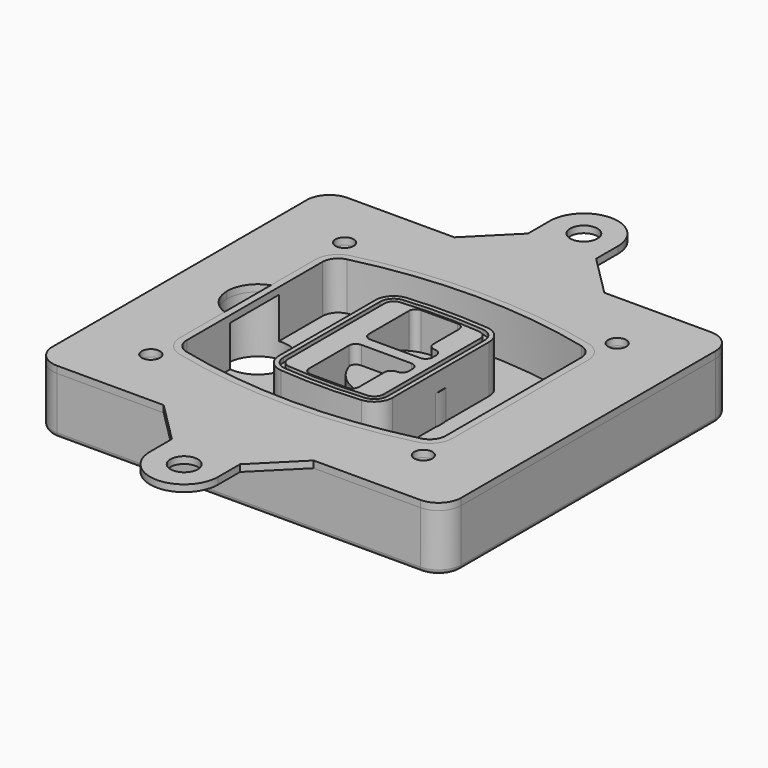
from build123d import *

# Parameters (mm, degrees)
F0_R      = 4
F1_DEPTH  = 25
F2_DEPTH  = 3
F3_DEPTH  = 18
F5_DEPTH  = 21
F6_DEPTH  = 2
F8_DEPTH  = 20
F9_DEPTH  = 16
F10_DEPTH = 25
F7_R      = 6
F7_R_2    = 4
F11_DEPTH = 6
F13_DEPTH = 9
F15_R     = 2
F16_R     = 6
F16_R_2   = 4
F17_DEPTH = 3


# Not quite as in the source:
# - a feature of the source that left no trace in its solid (it failed there, or was rolled back) is left out
# - a feature names something its author has since deleted; it is built from what else it names


with BuildPart() as f1:
    # F0 (on Top) → F1 (new body)
    with BuildSketch(Plane.XY):
        with BuildLine():
            ThreePointArc((-90, -70), (-87.0710678119, -77.0710678119), (-80, -80))
            Line((-80, -80), (80, -80))
            ThreePointArc((80, -80), (87.0710678119, -77.0710678119), (90, -70))
            Line((90, -70), (90, 70))
            ThreePointArc((90, 70), (87.0710678119, 77.0710678119), (80, 80))
            Line((80, 80), (-80, 80))
            ThreePointArc((-80, 80), (-87.0710678119, 77.0710678119), (-90, 70))
            Line((-90, 70), (-90, -70))
        make_face()
        with Locations((-60, -53.3333333333)):
            Circle(F0_R, mode=Mode.SUBTRACT)
        with Locations((60, -53.3333333333)):
            Circle(F0_R, mode=Mode.SUBTRACT)
        with Locations((-60, 53.3333333333)):
            Circle(F0_R, mode=Mode.SUBTRACT)
        with BuildLine():
            ThreePointArc((-64, 37.2990447398), (-61.0143011354, 45.9411029726), (-53.3306899286, 50.8970778549))
            ThreePointArc((-53.3306899286, 50.8970778549), (0, 57.3333333333), (53.3306899286, 50.8970778549))
            ThreePointArc((53.3306899286, 50.8970778549), (61.0143011354, 45.9411029726), (64, 37.2990447398))
            Line((64, 37.2990447398), (64, -37.2990447398))
            ThreePointArc((64, -37.2990447398), (61.0143011354, -45.9411029726), (53.3306899286, -50.8970778549))
            ThreePointArc((53.3306899286, -50.8970778549), (0, -57.3333333333), (-53.3306899286, -50.8970778549))
            ThreePointArc((-53.3306899286, -50.8970778549), (-61.0143011354, -45.9411029726), (-64, -37.2990447398))
            Line((-64, -37.2990447398), (-64, 37.2990447398))
        make_face(mode=Mode.SUBTRACT)
        with Locations((60, 53.3333333333)):
            Circle(F0_R, mode=Mode.SUBTRACT)
        with BuildLine():
            ThreePointArc((53.3306899286, 50.8970778549), (0, 57.3333333333), (-53.3306899286, 50.8970778549))
            ThreePointArc((-53.3306899286, 50.8970778549), (-61.0143011354, 45.9411029726), (-64, 37.2990447398))
            Line((-64, 37.2990447398), (-64, -37.2990447398))
            ThreePointArc((-64, -37.2990447398), (-61.0143011354, -45.9411029726), (-53.3306899286, -50.8970778549))
            ThreePointArc((-53.3306899286, -50.8970778549), (0, -57.3333333333), (53.3306899286, -50.8970778549))
            ThreePointArc((53.3306899286, -50.8970778549), (61.0143011354, -45.9411029726), (64, -37.2990447398))
            Line((64, -37.2990447398), (64, 37.2990447398))
            ThreePointArc((64, 37.2990447398), (61.0143011354, 45.9411029726), (53.3306899286, 50.8970778549))
        make_face()
        with BuildLine():
            Line((-60, -37.2990447398), (-60, 37.2990447398))
            ThreePointArc((-60, 37.2990447398), (-57.8673579538, 43.4719434775), (-52.3790642347, 47.0119255363))
            ThreePointArc((-52.3790642347, 47.0119255363), (0, 53.3333333333), (52.3790642347, 47.0119255363))
            ThreePointArc((52.3790642347, 47.0119255363), (57.8673579538, 43.4719434775), (60, 37.2990447398))
            Line((60, 37.2990447398), (60, -37.2990447398))
            ThreePointArc((60, -37.2990447398), (57.8673579538, -43.4719434775), (52.3790642347, -47.0119255363))
            ThreePointArc((52.3790642347, -47.0119255363), (0, -53.3333333333), (-52.3790642347, -47.0119255363))
            ThreePointArc((-52.3790642347, -47.0119255363), (-57.8673579538, -43.4719434775), (-60, -37.2990447398))
        make_face(mode=Mode.SUBTRACT)
        with BuildLine():
            ThreePointArc((-52.3790642347, 47.0119255363), (-57.8673579538, 43.4719434775), (-60, 37.2990447398))
            Line((-60, 37.2990447398), (-60, -37.2990447398))
            ThreePointArc((-60, -37.2990447398), (-57.8673579538, -43.4719434775), (-52.3790642347, -47.0119255363))
            ThreePointArc((-52.3790642347, -47.0119255363), (0, -53.3333333333), (52.3790642347, -47.0119255363))
            ThreePointArc((52.3790642347, -47.0119255363), (57.8673579538, -43.4719434775), (60, -37.2990447398))
            Line((60, -37.2990447398), (60, 37.2990447398))
            ThreePointArc((60, 37.2990447398), (57.8673579538, 43.4719434775), (52.3790642347, 47.0119255363))
            ThreePointArc((52.3790642347, 47.0119255363), (0, 53.3333333333), (-52.3790642347, 47.0119255363))
        make_face()
        with BuildLine():
            ThreePointArc((51.6653449643, 44.0980612973), (55.5071505677, 41.6200738562), (57, 37.2990447398))
            Line((57, 37.2990447398), (57, -37.2990447398))
            ThreePointArc((57, -37.2990447398), (55.5071505677, -41.6200738562), (51.6653449643, -44.0980612973))
            ThreePointArc((51.6653449643, -44.0980612973), (0, -50.3333333333), (-51.6653449643, -44.0980612973))
            ThreePointArc((-51.6653449643, -44.0980612973), (-55.5071505677, -41.6200738562), (-57, -37.2990447398))
            Line((-57, -37.2990447398), (-57, 37.2990447398))
            ThreePointArc((-57, 37.2990447398), (-55.5071505677, 41.6200738562), (-51.6653449643, 44.0980612973))
            ThreePointArc((-51.6653449643, 44.0980612973), (0, 50.3333333333), (51.6653449643, 44.0980612973))
        make_face(mode=Mode.SUBTRACT)
        with BuildLine():
            Line((57, -37.2990447398), (57, 37.2990447398))
            ThreePointArc((57, 37.2990447398), (55.5071505677, 41.6200738562), (51.6653449643, 44.0980612973))
            ThreePointArc((51.6653449643, 44.0980612973), (0, 50.3333333333), (-51.6653449643, 44.0980612973))
            ThreePointArc((-51.6653449643, 44.0980612973), (-55.5071505677, 41.6200738562), (-57, 37.2990447398))
            Line((-57, 37.2990447398), (-57, -37.2990447398))
            ThreePointArc((-57, -37.2990447398), (-55.5071505677, -41.6200738562), (-51.6653449643, -44.0980612973))
            ThreePointArc((-51.6653449643, -44.0980612973), (0, -50.3333333333), (51.6653449643, -44.0980612973))
            ThreePointArc((51.6653449643, -44.0980612973), (55.5071505677, -41.6200738562), (57, -37.2990447398))
        make_face()
    extrude(amount=-F1_DEPTH)

    # F0 (on Top) → F2 (join)
    with BuildSketch(Plane.XY):
        with BuildLine():
            ThreePointArc((-52.3790642347, 47.0119255363), (-57.8673579538, 43.4719434775), (-60, 37.2990447398))
            Line((-60, 37.2990447398), (-60, -37.2990447398))
            ThreePointArc((-60, -37.2990447398), (-57.8673579538, -43.4719434775), (-52.3790642347, -47.0119255363))
            ThreePointArc((-52.3790642347, -47.0119255363), (0, -53.3333333333), (52.3790642347, -47.0119255363))
            ThreePointArc((52.3790642347, -47.0119255363), (57.8673579538, -43.4719434775), (60, -37.2990447398))
            Line((60, -37.2990447398), (60, 37.2990447398))
            ThreePointArc((60, 37.2990447398), (57.8673579538, 43.4719434775), (52.3790642347, 47.0119255363))
            ThreePointArc((52.3790642347, 47.0119255363), (0, 53.3333333333), (-52.3790642347, 47.0119255363))
        make_face()
        with BuildLine():
            ThreePointArc((51.6653449643, 44.0980612973), (55.5071505677, 41.6200738562), (57, 37.2990447398))
            Line((57, 37.2990447398), (57, -37.2990447398))
            ThreePointArc((57, -37.2990447398), (55.5071505677, -41.6200738562), (51.6653449643, -44.0980612973))
            ThreePointArc((51.6653449643, -44.0980612973), (0, -50.3333333333), (-51.6653449643, -44.0980612973))
            ThreePointArc((-51.6653449643, -44.0980612973), (-55.5071505677, -41.6200738562), (-57, -37.2990447398))
            Line((-57, -37.2990447398), (-57, 37.2990447398))
            ThreePointArc((-57, 37.2990447398), (-55.5071505677, 41.6200738562), (-51.6653449643, 44.0980612973))
            ThreePointArc((-51.6653449643, 44.0980612973), (0, 50.3333333333), (51.6653449643, 44.0980612973))
        make_face(mode=Mode.SUBTRACT)
    extrude(amount=F2_DEPTH)

    # F0 (on Top) → F3 (cut)
    with BuildSketch(Plane.XY):
        with BuildLine():
            Line((57, -37.2990447398), (57, 37.2990447398))
            ThreePointArc((57, 37.2990447398), (55.5071505677, 41.6200738562), (51.6653449643, 44.0980612973))
            ThreePointArc((51.6653449643, 44.0980612973), (0, 50.3333333333), (-51.6653449643, 44.0980612973))
            ThreePointArc((-51.6653449643, 44.0980612973), (-55.5071505677, 41.6200738562), (-57, 37.2990447398))
            Line((-57, 37.2990447398), (-57, -37.2990447398))
            ThreePointArc((-57, -37.2990447398), (-55.5071505677, -41.6200738562), (-51.6653449643, -44.0980612973))
            ThreePointArc((-51.6653449643, -44.0980612973), (0, -50.3333333333), (51.6653449643, -44.0980612973))
            ThreePointArc((51.6653449643, -44.0980612973), (55.5071505677, -41.6200738562), (57, -37.2990447398))
        make_face()
    extrude(amount=-F3_DEPTH, mode=Mode.SUBTRACT)

    # F4 (on face) → F5 (join, through all)
    with BuildSketch(Plane.XY.offset(3)):
        with BuildLine():
            ThreePointArc((-25, -26.587695628), (-22.8992979869, -31.9912392117), (-17.7004291845, -34.5569740744))
            ThreePointArc((-17.7004291845, -34.5569740744), (0, -35.3333333333), (17.7004291845, -34.5569740744))
            ThreePointArc((17.7004291845, -34.5569740744), (22.8992979869, -31.9912392117), (25, -26.587695628))
            Line((25, -26.587695628), (25, 26.587695628))
            ThreePointArc((25, 26.587695628), (22.8992979869, 31.9912392117), (17.7004291845, 34.5569740744))
            ThreePointArc((17.7004291845, 34.5569740744), (0, 35.3333333333), (-17.7004291845, 34.5569740744))
            ThreePointArc((-17.7004291845, 34.5569740744), (-22.8992979869, 31.9912392117), (-25, 26.587695628))
            Line((-25, 26.587695628), (-25, -26.587695628))
        make_face()
        with BuildLine():
            ThreePointArc((17.5253218884, 32.5646544628), (21.4244734902, 30.6403533158), (23, 26.587695628))
            Line((23, 26.587695628), (23, -26.587695628))
            ThreePointArc((23, -26.587695628), (21.4244734902, -30.6403533158), (17.5253218884, -32.5646544628))
            ThreePointArc((17.5253218884, -32.5646544628), (0, -33.3333333333), (-17.5253218884, -32.5646544628))
            ThreePointArc((-17.5253218884, -32.5646544628), (-21.4244734902, -30.6403533158), (-23, -26.587695628))
            Line((-23, -26.587695628), (-23, 26.587695628))
            ThreePointArc((-23, 26.587695628), (-21.4244734902, 30.6403533158), (-17.5253218884, 32.5646544628))
            ThreePointArc((-17.5253218884, 32.5646544628), (0, 33.3333333333), (17.5253218884, 32.5646544628))
        make_face(mode=Mode.SUBTRACT)
        with BuildLine():
            Line((23, -26.587695628), (23, 26.587695628))
            ThreePointArc((23, 26.587695628), (21.4244734902, 30.6403533158), (17.5253218884, 32.5646544628))
            ThreePointArc((17.5253218884, 32.5646544628), (0, 33.3333333333), (-17.5253218884, 32.5646544628))
            ThreePointArc((-17.5253218884, 32.5646544628), (-21.4244734902, 30.6403533158), (-23, 26.587695628))
            Line((-23, 26.587695628), (-23, -26.587695628))
            ThreePointArc((-23, -26.587695628), (-21.4244734902, -30.6403533158), (-17.5253218884, -32.5646544628))
            ThreePointArc((-17.5253218884, -32.5646544628), (0, -33.3333333333), (17.5253218884, -32.5646544628))
            ThreePointArc((17.5253218884, -32.5646544628), (21.4244734902, -30.6403533158), (23, -26.587695628))
        make_face()
        with BuildLine():
            ThreePointArc((17.3502145923, 30.5723348512), (19.9496489934, 29.2894674198), (21, 26.587695628))
            Line((21, 26.587695628), (21, -26.587695628))
            ThreePointArc((21, -26.587695628), (19.9496489934, -29.2894674198), (17.3502145923, -30.5723348512))
            ThreePointArc((17.3502145923, -30.5723348512), (0, -31.3333333333), (-17.3502145923, -30.5723348512))
            ThreePointArc((-17.3502145923, -30.5723348512), (-19.9496489934, -29.2894674198), (-21, -26.587695628))
            Line((-21, -26.587695628), (-21, 26.587695628))
            ThreePointArc((-21, 26.587695628), (-19.9496489934, 29.2894674198), (-17.3502145923, 30.5723348512))
            ThreePointArc((-17.3502145923, 30.5723348512), (0, 31.3333333333), (17.3502145923, 30.5723348512))
        make_face(mode=Mode.SUBTRACT)
        with BuildLine():
            Line((21, -26.587695628), (21, 26.587695628))
            ThreePointArc((21, 26.587695628), (19.9496489934, 29.2894674198), (17.3502145923, 30.5723348512))
            ThreePointArc((17.3502145923, 30.5723348512), (0, 31.3333333333), (-17.3502145923, 30.5723348512))
            ThreePointArc((-17.3502145923, 30.5723348512), (-19.9496489934, 29.2894674198), (-21, 26.587695628))
            Line((-21, 26.587695628), (-21, -26.587695628))
            ThreePointArc((-21, -26.587695628), (-19.9496489934, -29.2894674198), (-17.3502145923, -30.5723348512))
            ThreePointArc((-17.3502145923, -30.5723348512), (0, -31.3333333333), (17.3502145923, -30.5723348512))
            ThreePointArc((17.3502145923, -30.5723348512), (19.9496489934, -29.2894674198), (21, -26.587695628))
        make_face()
        with BuildLine():
            Line((-8, -2.5), (14, -2.5))
            ThreePointArc((14, -2.5), (16.1213203436, -3.3786796564), (17, -5.5))
            Line((17, -5.5), (17, -7.5))
            ThreePointArc((17, -7.5), (16.1213203436, -9.6213203436), (14, -10.5))
            ThreePointArc((14, -10.5), (11.8786796564, -11.3786796564), (11, -13.5))
            Line((11, -13.5), (11, -27.5))
            ThreePointArc((11, -27.5), (10.1213203436, -29.6213203436), (8, -30.5))
            Line((8, -30.5), (-8, -30.5))
            ThreePointArc((-8, -30.5), (-10.1213203436, -29.6213203436), (-11, -27.5))
            Line((-11, -27.5), (-11, -5.5))
            ThreePointArc((-11, -5.5), (-10.1213203436, -3.3786796564), (-8, -2.5))
        make_face(mode=Mode.SUBTRACT)
        with BuildLine():
            ThreePointArc((-8, 2.5), (-10.1213203436, 3.3786796564), (-11, 5.5))
            Line((-11, 5.5), (-11, 27.5))
            ThreePointArc((-11, 27.5), (-10.1213203436, 29.6213203436), (-8, 30.5))
            Line((-8, 30.5), (8, 30.5))
            ThreePointArc((8, 30.5), (10.1213203436, 29.6213203436), (11, 27.5))
            Line((11, 27.5), (11, 13.5))
            ThreePointArc((11, 13.5), (11.8786796564, 11.3786796564), (14, 10.5))
            ThreePointArc((14, 10.5), (16.1213203436, 9.6213203436), (17, 7.5))
            Line((17, 7.5), (17, 5.5))
            ThreePointArc((17, 5.5), (16.1213203436, 3.3786796564), (14, 2.5))
            Line((14, 2.5), (-8, 2.5))
        make_face(mode=Mode.SUBTRACT)
    extrude(amount=-F5_DEPTH)

    # F4 (on face) → F6 (cut)
    with BuildSketch(Plane.XY.offset(3)):
        with BuildLine():
            Line((23, -26.587695628), (23, 26.587695628))
            ThreePointArc((23, 26.587695628), (21.4244734902, 30.6403533158), (17.5253218884, 32.5646544628))
            ThreePointArc((17.5253218884, 32.5646544628), (0, 33.3333333333), (-17.5253218884, 32.5646544628))
            ThreePointArc((-17.5253218884, 32.5646544628), (-21.4244734902, 30.6403533158), (-23, 26.587695628))
            Line((-23, 26.587695628), (-23, -26.587695628))
            ThreePointArc((-23, -26.587695628), (-21.4244734902, -30.6403533158), (-17.5253218884, -32.5646544628))
            ThreePointArc((-17.5253218884, -32.5646544628), (0, -33.3333333333), (17.5253218884, -32.5646544628))
            ThreePointArc((17.5253218884, -32.5646544628), (21.4244734902, -30.6403533158), (23, -26.587695628))
        make_face()
        with BuildLine():
            ThreePointArc((17.3502145923, 30.5723348512), (19.9496489934, 29.2894674198), (21, 26.587695628))
            Line((21, 26.587695628), (21, -26.587695628))
            ThreePointArc((21, -26.587695628), (19.9496489934, -29.2894674198), (17.3502145923, -30.5723348512))
            ThreePointArc((17.3502145923, -30.5723348512), (0, -31.3333333333), (-17.3502145923, -30.5723348512))
            ThreePointArc((-17.3502145923, -30.5723348512), (-19.9496489934, -29.2894674198), (-21, -26.587695628))
            Line((-21, -26.587695628), (-21, 26.587695628))
            ThreePointArc((-21, 26.587695628), (-19.9496489934, 29.2894674198), (-17.3502145923, 30.5723348512))
            ThreePointArc((-17.3502145923, 30.5723348512), (0, 31.3333333333), (17.3502145923, 30.5723348512))
        make_face(mode=Mode.SUBTRACT)
    extrude(amount=-F6_DEPTH, mode=Mode.SUBTRACT)

    # F7 (on face) → F8 (join)
    with BuildSketch(Plane(origin=(0, 0, -25), x_dir=(1, 0, 0), z_dir=(0, 0, -1))):
        with BuildLine():
            ThreePointArc((-6.71157564, 0), (6.7567035675, 13.4682792075), (20.224982775, 0))
            Line((20.224982775, 0), (25.224982775, 0))
            ThreePointArc((25.224982775, 0), (6.7567035675, 18.4682792075), (-11.71157564, 0))
            Line((-11.71157564, 0), (-6.71157564, 0))
        make_face()
        with BuildLine():
            Line((-6.71157564, 0), (20.224982775, 0))
            ThreePointArc((20.224982775, 0), (6.7567035675, 13.4682792075), (-6.71157564, 0))
        make_face()
        with BuildLine():
            ThreePointArc((-6.71157564, 0), (6.7567035675, -13.4682792075), (20.224982775, 0))
            Line((20.224982775, 0), (-6.71157564, 0))
        make_face()
        with BuildLine():
            Line((25.224982775, 0), (20.224982775, 0))
            ThreePointArc((20.224982775, 0), (6.7567035675, -13.4682792075), (-6.71157564, 0))
            Line((-6.71157564, 0), (-11.71157564, 0))
            ThreePointArc((-11.71157564, 0), (6.7567035675, -18.4682792075), (25.224982775, 0))
        make_face()
    extrude(amount=-F8_DEPTH)

    # F7 (on face) → F9 (cut)
    with BuildSketch(Plane(origin=(0, 0, -25), x_dir=(1, 0, 0), z_dir=(0, 0, -1))):
        with BuildLine():
            Line((-6.71157564, 0), (20.224982775, 0))
            ThreePointArc((20.224982775, 0), (6.7567035675, 13.4682792075), (-6.71157564, 0))
        make_face()
        with BuildLine():
            ThreePointArc((-6.71157564, 0), (6.7567035675, -13.4682792075), (20.224982775, 0))
            Line((20.224982775, 0), (-6.71157564, 0))
        make_face()
    extrude(amount=-F9_DEPTH, mode=Mode.SUBTRACT)

    # F7 (on face) → F10 (cut)
    with BuildSketch(Plane(origin=(0, 0, -25), x_dir=(1, 0, 0), z_dir=(0, 0, -1))):
        with BuildLine():
            Line((-69.0318229325, 0), (-42.0952645175, 0))
            ThreePointArc((-42.0952645175, 0), (-55.563543725, 13.4682792075), (-69.0318229325, 0))
        make_face()
        with BuildLine():
            ThreePointArc((-69.0318229325, 0), (-55.563543725, -13.4682792075), (-42.0952645175, 0))
            Line((-42.0952645175, 0), (-69.0318229325, 0))
        make_face()
    extrude(amount=-F10_DEPTH, mode=Mode.SUBTRACT)

    # F7 (on face) → F11 (cut)
    with BuildSketch(Plane(origin=(0, 0, -25), x_dir=(1, 0, 0), z_dir=(0, 0, -1))):
        with Locations((60, -53.3333333333)):
            Circle(F7_R)
        with Locations((60, -53.3333333333)):
            Circle(F7_R_2, mode=Mode.SUBTRACT)
        with Locations((-60, -53.3333333333)):
            Circle(F7_R)
        with Locations((-60, -53.3333333333)):
            Circle(F7_R_2, mode=Mode.SUBTRACT)
        with Locations((-60, 53.3333333333)):
            Circle(F7_R)
        with Locations((-60, 53.3333333333)):
            Circle(F7_R_2, mode=Mode.SUBTRACT)
        with Locations((60, 53.3333333333)):
            Circle(F7_R)
        with Locations((60, 53.3333333333)):
            Circle(F7_R_2, mode=Mode.SUBTRACT)
    extrude(amount=-F11_DEPTH, mode=Mode.SUBTRACT)

    # F12 (on face) → F13 (cut, through all)
    with BuildSketch(Plane(origin=(0, 0, -9), x_dir=(1, 0, 0), z_dir=(0, 0, -1))):
        with BuildLine():
            ThreePointArc((20.224982775, 0), (20.1663399806, 1.2554664788), (19.9909222755, 2.5))
            Line((19.9909222755, 2.5), (14, 2.5))
            ThreePointArc((14, 2.5), (16.1213203436, 3.3786796564), (17, 5.5))
            Line((17, 5.5), (17, 7.5))
            ThreePointArc((17, 7.5), (16.1213203436, 9.6213203436), (14, 10.5))
            ThreePointArc((14, 10.5), (12.1627255951, 11.1284134507), (11.0951631559, 12.750384826))
            ThreePointArc((11.0951631559, 12.750384826), (11.0476113807, 12.7664660322), (11, 12.7823698976))
            Line((11, 12.7823698976), (11, -12.7823698976))
            ThreePointArc((11, -12.7823698976), (11.0476113807, -12.7664660322), (11.0951631559, -12.750384826))
            ThreePointArc((11.0951631559, -12.750384826), (12.1627255951, -11.1284134507), (14, -10.5))
            ThreePointArc((14, -10.5), (16.1213203436, -9.6213203436), (17, -7.5))
            Line((17, -7.5), (17, -5.5))
            ThreePointArc((17, -5.5), (16.1213203436, -3.3786796564), (14, -2.5))
            Line((14, -2.5), (19.9909222755, -2.5))
            ThreePointArc((19.9909222755, -2.5), (20.1663399806, -1.2554664788), (20.224982775, 0))
        make_face()
    extrude(amount=F13_DEPTH, mode=Mode.SUBTRACT)

    # F15
    f15_edges = [f1.edges().sort_by_distance(p)[0] for p in [
        (0, -80, -25),
        (-87.071068, -77.071068, -25),
        (-90, 0, -25),
        (-87.071068, 77.071068, -25),
        (87.071068, -77.071068, -25),
        (0, 80, -25),
        (90, 0, -25),
        (87.071068, 77.071068, -25),
    ]]
    fillet(f15_edges, radius=F15_R)


with BuildPart() as f17:
    # F16 (on face) → F17 (new body, through all)
    with BuildSketch(Plane.XY):
        with BuildLine():
            ThreePointArc((15, 110), (0, 125), (-15, 110))
            Line((-15, 110), (-15, 98))
            Line((-15, 98), (-33, 80))
            Line((-33, 80), (33, 80))
            Line((33, 80), (15, 98))
            Line((15, 98), (15, 110))
        make_face()
        with Locations((0, 110)):
            Circle(F16_R, mode=Mode.SUBTRACT)
        with BuildLine():
            Line((33, 80), (-33, 80))
            Line((-33, 80), (-80, 80))
            ThreePointArc((-80, 80), (-87.0710678119, 77.0710678119), (-90, 70))
            Line((-90, 70), (-90, -70))
            ThreePointArc((-90, -70), (-87.0710678119, -77.0710678119), (-80, -80))
            Line((-80, -80), (-33, -80))
            Line((-33, -80), (33, -80))
            Line((33, -80), (80, -80))
            ThreePointArc((80, -80), (87.0710678119, -77.0710678119), (90, -70))
            Line((90, -70), (90, 70))
            ThreePointArc((90, 70), (87.0710678119, 77.0710678119), (80, 80))
            Line((80, 80), (33, 80))
        make_face()
        with Locations((-60, -53.3333333333)):
            Circle(F16_R_2, mode=Mode.SUBTRACT)
        with Locations((60, -53.3333333333)):
            Circle(F16_R_2, mode=Mode.SUBTRACT)
        with Locations((-60, 53.3333333333)):
            Circle(F16_R_2, mode=Mode.SUBTRACT)
        with BuildLine():
            Line((-60, 12.7166190685), (-60, 37.2990447398))
            ThreePointArc((-60, 37.2990447398), (-57.8673579538, 43.4719434775), (-52.3790642347, 47.0119255363))
            ThreePointArc((-52.3790642347, 47.0119255363), (0, 53.3333333333), (52.3790642347, 47.0119255363))
            ThreePointArc((52.3790642347, 47.0119255363), (57.8673579538, 43.4719434775), (60, 37.2990447398))
            Line((60, 37.2990447398), (60, -37.2990447398))
            ThreePointArc((60, -37.2990447398), (57.8673579538, -43.4719434775), (52.3790642347, -47.0119255363))
            ThreePointArc((52.3790642347, -47.0119255363), (0, -53.3333333333), (-52.3790642347, -47.0119255363))
            ThreePointArc((-52.3790642347, -47.0119255363), (-57.8673579538, -43.4719434775), (-60, -37.2990447398))
            Line((-60, -37.2990447398), (-60, -12.7166190685))
            ThreePointArc((-60, -12.7166190685), (-66.5441169481, -7.798817635), (-69.0318229325, 0))
            ThreePointArc((-69.0318229325, 0), (-66.5441169481, 7.798817635), (-60, 12.7166190685))
        make_face(mode=Mode.SUBTRACT)
        with Locations((60, 53.3333333333)):
            Circle(F16_R_2, mode=Mode.SUBTRACT)
        with BuildLine():
            Line((33, -80), (-33, -80))
            Line((-33, -80), (-15, -98))
            Line((-15, -98), (-15, -110))
            ThreePointArc((-15, -110), (0, -125), (15, -110))
            Line((15, -110), (15, -98))
            Line((15, -98), (33, -80))
        make_face()
        with Locations((0, -110)):
            Circle(F16_R, mode=Mode.SUBTRACT)
    extrude(amount=F17_DEPTH)


solid = Compound([f1.part, f17.part])
